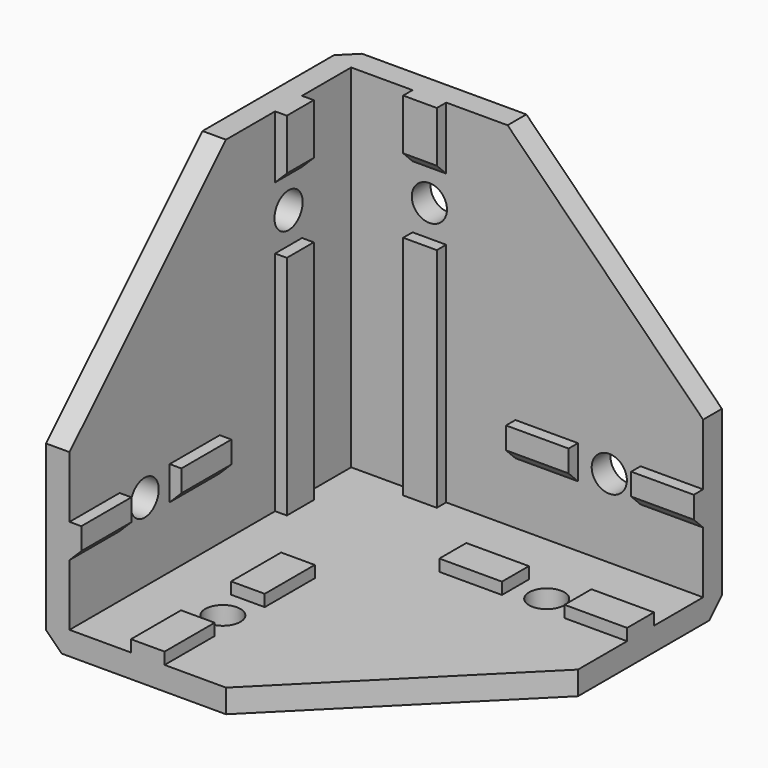
from build123d import *

# Parameters (mm, degrees)
F0_R     = 2.25
F0_W     = 4.3
F0_H     = 8
F0_W_2   = 8
F0_H_2   = 4.3
F1_DEPTH = 3
F2_DEPTH = 45
F3_DEPTH = 1.5
F4_R     = 2.25
F5_DEPTH = 12.5
F4_W     = 4.3
F4_H     = 8
F4_H_2   = 21
F4_W_2   = 8
F4_H_3   = 4.3
F6_DEPTH = 1.5
F7_SIZE  = 1.49999
F9_SIZE  = 2


# Not quite as in the source:
# - a fillet or chamfer is up to 0.001 mm smaller than in the source, because OpenCascade refuses the exact size
# - a pattern or mirror of a feature is missing from the dataset's text; its kind, count and spacing are read off the source's solid


with BuildPart() as f1:
    # F0 (on Top) → F1 (new body)
    with BuildSketch(Plane.XY):
        Polygon((0, -45), (0, 0), (45, 0), (45, 3), (-3, 3), (-3, -45), align=None)
        Polygon((45, 0), (0, 0), (0, -45), (7.85, -45), (7.85, -37), (12.15, -37), (12.15, -45), (20, -45), (45, -20), (45, -12.15), (37, -12.15), (37, -7.85), (45, -7.85), align=None)
        with Locations((10, -33)):
            Circle(F0_R, mode=Mode.SUBTRACT)
        with Locations((10, -25)):
            Rectangle(F0_W, F0_H, mode=Mode.SUBTRACT)
        with Locations((25, -10)):
            Rectangle(F0_W_2, F0_H_2, mode=Mode.SUBTRACT)
        with Locations((33, -10)):
            Circle(F0_R, mode=Mode.SUBTRACT)
        with Locations((25, -10)):
            Rectangle(F0_W_2, F0_H_2)
        with Locations((41, -10)):
            Rectangle(F0_W_2, F0_H_2)
        with Locations((10, -25)):
            Rectangle(F0_W, F0_H)
        with Locations((10, -41)):
            Rectangle(F0_W, F0_H)
    extrude(amount=-F1_DEPTH)

    # F0 (on Top) → F2 (join)
    with BuildSketch(Plane.XY):
        Polygon((0, -45), (0, 0), (45, 0), (45, 3), (-3, 3), (-3, -45), align=None)
    extrude(amount=F2_DEPTH)

    # F0 (on Top) → F3 (join)
    with BuildSketch(Plane.XY):
        with Locations((10, -25)):
            Rectangle(F0_W, F0_H)
        with Locations((10, -41)):
            Rectangle(F0_W, F0_H)
        with Locations((25, -10)):
            Rectangle(F0_W_2, F0_H_2)
        with Locations((41, -10)):
            Rectangle(F0_W_2, F0_H_2)
    extrude(amount=F3_DEPTH)

    # F4 (on face) → F5 (cut, symmetric)
    with BuildSketch(Plane.YZ):
        Polygon((-45, 20), (-20, 45), (-45, 45), align=None)
        with Locations((-10, 33)):
            Circle(F4_R)
        with Locations((-33, 10)):
            Circle(F4_R)
    f5 = extrude(amount=F5_DEPTH, both=True, mode=Mode.SUBTRACT)

    # F5_copies: F5 across plane
    add(f5.mirror(Plane(origin=(0, 0, 0), x_dir=(0.7071067812, -0.7071067812, 0), z_dir=(0.7071067812, 0.7071067812, 0))), mode=Mode.SUBTRACT)

    # F4 (on face) → F6 (join)
    with BuildSketch(Plane.YZ):
        with Locations((-10, 41)):
            Rectangle(F4_W, F4_H)
        with Locations((-10, 25)):
            Rectangle(F4_W, F4_H)
        with Locations((-10, 10.5)):
            Rectangle(F4_W, F4_H_2)
        with Locations((-25, 10)):
            Rectangle(F4_W_2, F4_H_3)
        with Locations((-41, 10)):
            Rectangle(F4_W_2, F4_H_3)
    f6 = extrude(amount=F6_DEPTH)

    # F6_copies: F6 across plane
    add(f6.mirror(Plane(origin=(0, 0, 0), x_dir=(0.7071067812, -0.7071067812, 0), z_dir=(0.7071067812, 0.7071067812, 0))))

    # F7 (size 1.5 in the source; OpenCascade refuses exactly that, so slightly less here)
    f7_edges = [f1.edges().sort_by_distance(p)[0] for p in [
        (1.5, -41, 7.85),
        (1.5, -25, 7.85),
        (1.5, -10, 37),
        (41, -1.5, 7.85),
        (10, -1.5, 37),
        (25, -1.5, 7.85),
    ]]
    chamfer(f7_edges, length=F7_SIZE)

    # F9
    f9_edges = [f1.edges().sort_by_distance(p)[0] for p in [
        (-3, 3, 21),
        (-3, -21, -3),
        (21, 3, -3),
    ]]
    chamfer(f9_edges, length=F9_SIZE)


solid = f1.part
